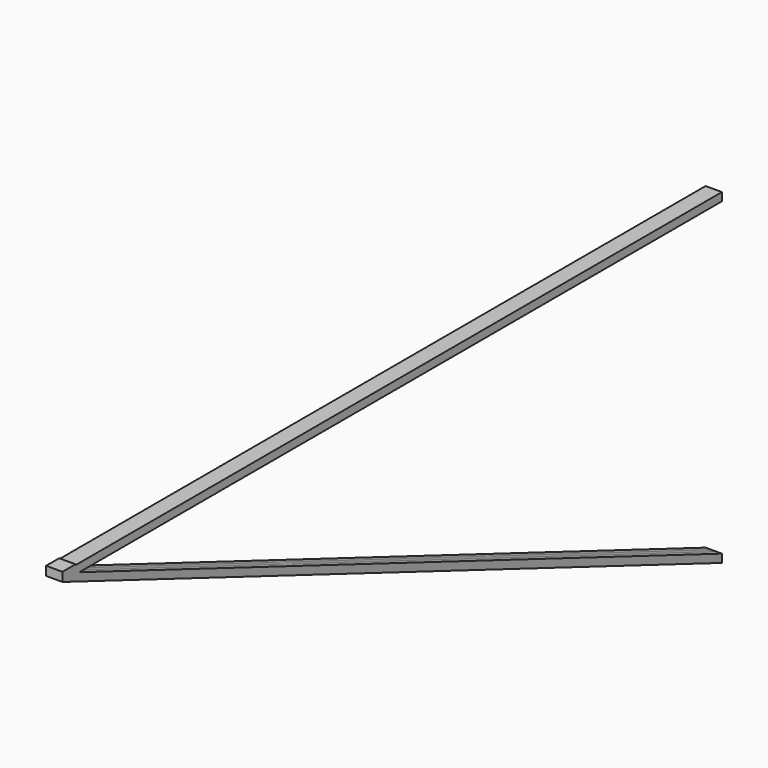
from build123d import *

# Parameters (mm, degrees)
F1_DEPTH  = 505
F2_DEPTH  = 500.5
F4_DEPTH  = 10
F5_DEPTH  = 10
F7_DEPTH  = 3.5
F8_W      = 10
F8_H      = 10
F10_DEPTH = 0.5
F11_DEPTH = 3.5
F12_W     = 3
F12_H     = 158.2
F12_H_2   = 149.0364306936
F12_H_3   = 168.1512820513
F13_DEPTH = 3
F14_W     = 3
F14_H     = 180.2518238002
F14_H_2   = 163.2489754916
F14_H_3   = 161.2561033061
F15_DEPTH = 3
F16_DEPTH = 40
F17_W     = 5.5675039161
F17_H     = 3.688506484
F18_DEPTH = 25
F19_DEPTH = 25


with BuildPart() as f1:
    # F0 (on Front) → F1 (new body)
    with BuildSketch(Plane.XZ):
        Polygon((5, 0), (0, 0), (-5, 0), (-5, -200), (5, -200), align=None)
    extrude(amount=F1_DEPTH)

    # F0 (on Front) → F2 (join)
    with BuildSketch(Plane.XZ):
        Polygon((5, 0), (0, 0), (-5, 0), (-5, -200), (5, -200), align=None)
    extrude(amount=F2_DEPTH)

    # F3 (on face) → F4 (cut, through all)
    with BuildSketch(Plane(origin=(-5, 0, 0), x_dir=(0, -1, 0), z_dir=(-1, 0, 0))):
        Polygon((328.8512820513, -65.3208171387), (328.8512820513, -5), (179.8148513577, -5), align=None)
        Polygon((173.1512820513, -128.1396039604), (325.4411393395, -69.334609562), (173.1512820513, -7.6970046434), align=None)
        Polygon((168.1512820513, -5), (0, -5), (0, -195), (168.1512820513, -130.0702970297), align=None)
        Polygon((333.8512820513, -66.0871287129), (492.0512820513, -5), (333.8512820513, -5), align=None)
    extrude(amount=-F4_DEPTH, mode=Mode.SUBTRACT)

    # F3 (on face) → F5 (cut, through all)
    with BuildSketch(Plane(origin=(-5, 0, 0), x_dir=(0, -1, 0), z_dir=(-1, 0, 0))):
        Polygon((505, -200), (505, -5), (331.3512820513, -72.0524752475), (0, -200), align=None)
    extrude(amount=-F5_DEPTH, mode=Mode.SUBTRACT)

    # F6 (on face) → F7 (cut)
    with BuildSketch(Plane(origin=(-5, 0, 0), x_dir=(0, -1, 0), z_dir=(-1, 0, 0))):
        Polygon((179.8148513577, -5), (168.1512820513, -5), (168.1512820513, -130.0702970297), (173.1512820513, -128.1396039604), (173.1512820513, -7.6970046434), (325.4411393395, -69.334609562), (333.8512820513, -66.0871287129), (333.8512820513, -5), (328.8512820513, -5), (328.8512820513, -65.3208171387), align=None)
    extrude(amount=-F7_DEPTH, mode=Mode.SUBTRACT)

    # F8 (on face) → F10 (join)
    with BuildSketch(Plane.XY):
        with Locations((0, -500)):
            Rectangle(F8_W, F8_H)
    extrude(amount=F10_DEPTH)

    # F9 (on face) → F11 (cut)
    with BuildSketch(Plane.YZ.offset(5)):
        Polygon((-173.1512820513, -7.6970046434), (-173.1512820513, -128.1396039604), (-168.1512820513, -130.0702970297), (-168.1512820513, -5), (-179.8148513577, -5), (-328.8512820513, -65.3208171387), (-328.8512820513, -5), (-333.8512820513, -5), (-333.8512820513, -66.0871287129), (-325.4411393395, -69.334609562), align=None)
    extrude(amount=-F11_DEPTH, mode=Mode.SUBTRACT)

    # F12 (on face) → F13 (join)
    with BuildSketch(Plane(origin=(0, 0, -5), x_dir=(1, 0, 0), z_dir=(0, 0, -1))):
        with Locations((0, 412.9512820513)):
            Rectangle(F12_W, F12_H)
        with Locations((0, 254.3330667045)):
            Rectangle(F12_W, F12_H_2)
        with Locations((0, 84.0756410256)):
            Rectangle(F12_W, F12_H_3)
    extrude(amount=F13_DEPTH)

    # F14 (on face) → F15 (join)
    with BuildSketch(Plane(origin=(0, -65.5267872377, -169.6975772053), x_dir=(1, 0, 0), z_dir=(0, 0.3602166214, 0.9328686862))):
        with Locations((0, -19.8836707273)):
            Rectangle(F14_W, F14_H)
        with Locations((0, -196.9938815385)):
            Rectangle(F14_W, F14_H_2)
        with Locations((0, -368.2617762991)):
            Rectangle(F14_W, F14_H_3)
    extrude(amount=F15_DEPTH)

    # F16 (add): a face of the model
    f16_faces = [f1.faces().sort_by_distance(p)[0] for p in [
        (0, -167.6109571192, -128.6709940004),
    ]]
    extrude(f16_faces, amount=F16_DEPTH)

    # F17 (on face) → F18 (cut)
    with BuildSketch(Plane(origin=(0, 0, 0), x_dir=(-1, 0, 0), z_dir=(0, 1, 0))):
        with Locations((-0.283751958, -193.155746758)):
            Rectangle(F17_W, F17_H)
    extrude(amount=F18_DEPTH, mode=Mode.SUBTRACT)

    # F19 (cut): a face of the model
    f19_faces = [f1.faces().sort_by_distance(p)[0] for p in [
        (-1.5, -84.0756410256, -7.4725396089),
    ]]
    extrude(f19_faces, amount=-F19_DEPTH, mode=Mode.SUBTRACT)


solid = f1.part
